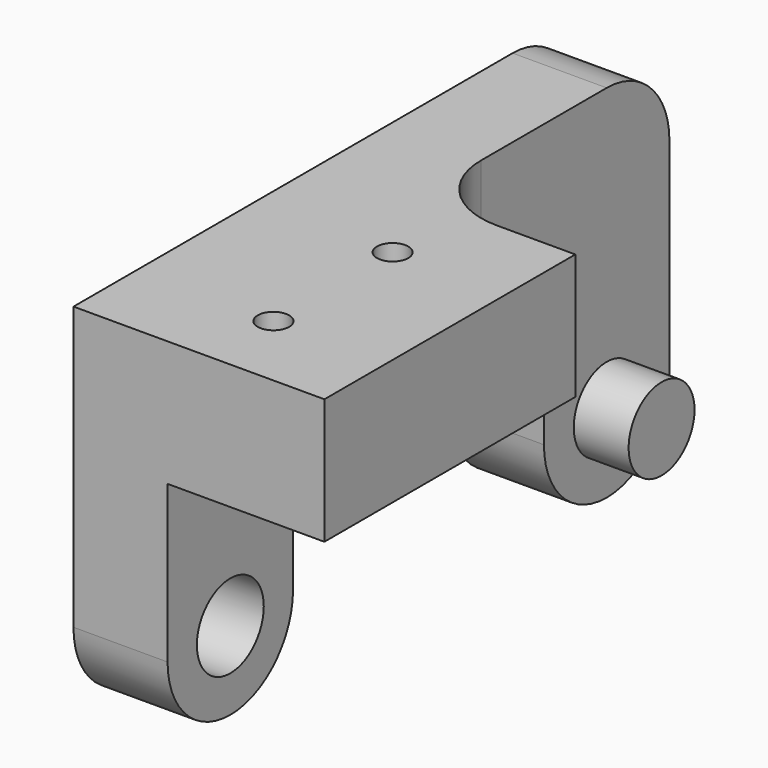
from build123d import *

# Parameters (mm, degrees)
F0_R     = 2.667
F0_R_2   = 2.625
F2_DEPTH = 6
F3_DEPTH = 3.5
F4_DEPTH = 4
F5_DEPTH = 10
F1_R     = 1
F6_DEPTH = 18.001
F7_R     = 4.99999


# Not quite as in the source:
# - a fillet or chamfer is up to 0.001 mm smaller than in the source, because OpenCascade refuses the exact size


with BuildPart() as f2:
    # F0 (on Right) → F2 (new body)
    with BuildSketch(Plane.YZ):
        Polygon((7.0520542562, 18), (-12.9479457438, 18), (-12.9479457438, 10), (-2.9479457438, 10), (7.0520542562, 10), align=None)
        with BuildLine():
            Line((22.0520542562, 18), (7.0520542562, 18))
            Line((7.0520542562, 18), (7.0520542562, 10))
            Line((7.0520542562, 10), (17.0520542562, 10))
            Line((17.0520542562, 10), (27.0520542562, 10))
            Line((27.0520542562, 10), (27.0520542562, 13))
            ThreePointArc((27.0520542562, 13), (25.5875881621, 16.5355339059), (22.0520542562, 18))
        make_face()
        with BuildLine():
            Line((-2.9479457438, 10), (-12.9479457438, 10))
            Line((-12.9479457438, 10), (-12.9479457438, 0))
            ThreePointArc((-12.9479457438, 0), (-11.4834796497, -3.5355339059), (-7.9479457438, -5))
            ThreePointArc((-7.9479457438, -5), (-4.4124118379, -3.5355339059), (-2.9479457438, 0))
            Line((-2.9479457438, 0), (-2.9479457438, 10))
        make_face()
        with Locations((-7.9479457438, 0)):
            Circle(F0_R, mode=Mode.SUBTRACT)
        with BuildLine():
            Line((27.0520542562, 10), (17.0520542562, 10))
            Line((17.0520542562, 10), (17.0520542562, 0))
            ThreePointArc((17.0520542562, 0), (18.5165203503, -3.5355339059), (22.0520542562, -5))
            ThreePointArc((22.0520542562, -5), (25.5875881621, -3.5355339059), (27.0520542562, 0))
            Line((27.0520542562, 0), (27.0520542562, 10))
        make_face()
        with Locations((22.0520542562, 0)):
            Circle(F0_R_2, mode=Mode.SUBTRACT)
        with Locations((-7.9479457438, 0)):
            Circle(F0_R)
        with Locations((22.0520542562, 0)):
            Circle(F0_R_2)
    extrude(amount=-F2_DEPTH)

    # F0 (on Right) → F3 (join)
    with BuildSketch(Plane.YZ):
        with Locations((22.0520542562, 0)):
            Circle(F0_R_2)
    extrude(amount=F3_DEPTH)

    # F0 (on Right) → F4 (cut)
    with BuildSketch(Plane.YZ):
        with Locations((-7.9479457438, 0)):
            Circle(F0_R)
    extrude(amount=-F4_DEPTH, mode=Mode.SUBTRACT)

    # F0 (on Right) → F5 (join)
    with BuildSketch(Plane.YZ):
        Polygon((7.0520542562, 18), (-12.9479457438, 18), (-12.9479457438, 10), (-2.9479457438, 10), (7.0520542562, 10), align=None)
    extrude(amount=F5_DEPTH)

    # F1 (on Top) → F6 (cut, through all)
    with BuildSketch(Plane.XY):
        with Locations((2.75, 1.5520542562)):
            Circle(F1_R)
        with Locations((2.75, -7.9479457438)):
            Circle(F1_R)
    extrude(amount=F6_DEPTH, mode=Mode.SUBTRACT)

    # F7 (radius 5 in the source; OpenCascade refuses exactly that, so slightly less here)
    f7_edges = [f2.edges().sort_by_distance(p)[0] for p in [
        (0, 7.052054, 14),
        (-3, -2.947946, 10),
        (-3, 17.052054, 10),
    ]]
    fillet(f7_edges, radius=F7_R)


solid = f2.part
